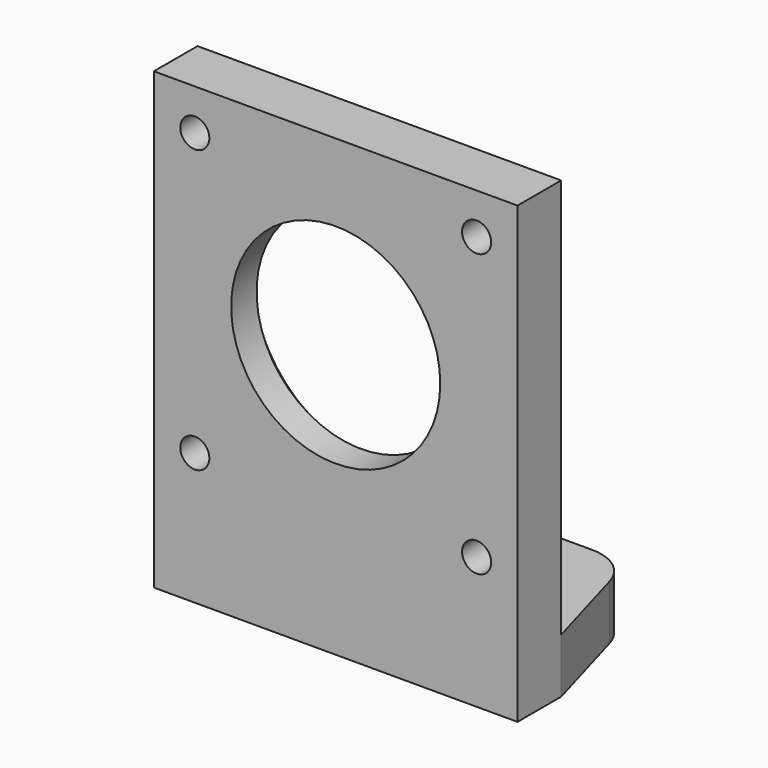
from build123d import *

# Parameters (mm, degrees)
F1_W     = 12
F1_H     = 14
F1_R     = 2.6
F2_DEPTH = 6
F3_DEPTH = 50
F4_R     = 11.5
F4_R_2   = 1.6
F5_DEPTH = 20.001
F7_R     = 5
F8_SIZE  = 2.5


with BuildPart() as f2:
    # F1 (on Top) → F2 (new body)
    with BuildSketch(Plane.XY):
        with Locations((-10, 30.4999971617)):
            Rectangle(F1_W, F1_H)
        with Locations((-10, 30.4999971617)):
            Circle(F1_R, mode=Mode.SUBTRACT)
        with BuildLine():
            Line((10, 33.0999971617), (10, 37.4999971617))
            Line((10, 37.4999971617), (4, 37.4999971617))
            Line((4, 37.4999971617), (4, 30.4999971617))
            Line((4, 30.4999971617), (7.4, 30.4999971617))
            ThreePointArc((7.4, 30.4999971617), (8.1615223689, 32.3384747928), (10, 33.0999971617))
        make_face()
        with BuildLine():
            Line((16, 30.4999971617), (16, 37.4999971617))
            Line((16, 37.4999971617), (10, 37.4999971617))
            Line((10, 37.4999971617), (10, 33.0999971617))
            ThreePointArc((10, 33.0999971617), (11.8384776311, 32.3384747928), (12.6, 30.4999971617))
            Line((12.6, 30.4999971617), (16, 30.4999971617))
        make_face()
        with BuildLine():
            Line((10, 23.4999971617), (16, 23.4999971617))
            Line((16, 23.4999971617), (16, 30.4999971617))
            Line((16, 30.4999971617), (12.6, 30.4999971617))
            ThreePointArc((12.6, 30.4999971617), (11.8384776311, 28.6615195306), (10, 27.8999971617))
            Line((10, 27.8999971617), (10, 23.4999971617))
        make_face()
        with BuildLine():
            Line((4, 23.4999971617), (10, 23.4999971617))
            Line((10, 23.4999971617), (10, 27.8999971617))
            ThreePointArc((10, 27.8999971617), (8.1615223689, 28.6615195306), (7.4, 30.4999971617))
            Line((7.4, 30.4999971617), (4, 30.4999971617))
            Line((4, 30.4999971617), (4, 23.4999971617))
        make_face()
        Polygon((-16, 37.4999971617), (-20, 23.4999971617), (-16, 23.4999971617), align=None)
        Polygon((-4, 37.4999971617), (-4, 23.4999971617), (4, 23.4999971617), (4, 30.4999971617), (4, 37.4999971617), align=None)
        Polygon((16, 23.4999971617), (20, 23.4999971617), (16, 37.4999971617), (16, 30.4999971617), align=None)
    extrude(amount=F2_DEPTH)

    # F1 (on Top) → F3 (join)
    with BuildSketch(Plane.XY):
        Polygon((-20, 23.4999971617), (-20, 17.4999971617), (20, 17.4999971617), (20, 23.4999971617), (16, 23.4999971617), (10, 23.4999971617), (4, 23.4999971617), (-4, 23.4999971617), (-16, 23.4999971617), align=None)
    extrude(amount=F3_DEPTH)

    # F4 (on face) → F5 (cut, through all)
    with BuildSketch(Plane.XZ.offset(-17.4999971617)):
        with Locations((0, 30)):
            Circle(F4_R)
        with Locations((-15.5, 45.5)):
            Circle(F4_R_2)
        with Locations((-15.5, 14.5)):
            Circle(F4_R_2)
        with Locations((15.5, 14.5)):
            Circle(F4_R_2)
        with Locations((15.5, 45.5)):
            Circle(F4_R_2)
    extrude(amount=-F5_DEPTH, mode=Mode.SUBTRACT)

    # F7
    f7_edges = [f2.edges().sort_by_distance(p)[0] for p in [
        (16, 37.499997, 3),
        (-16, 37.499997, 3),
    ]]
    fillet(f7_edges, radius=F7_R)

    # F8
    f8_edges = [f2.edges().sort_by_distance(p)[0] for p in [
        (-11.5, 23.499997, 30),
    ]]
    chamfer(f8_edges, length=F8_SIZE)


solid = f2.part
